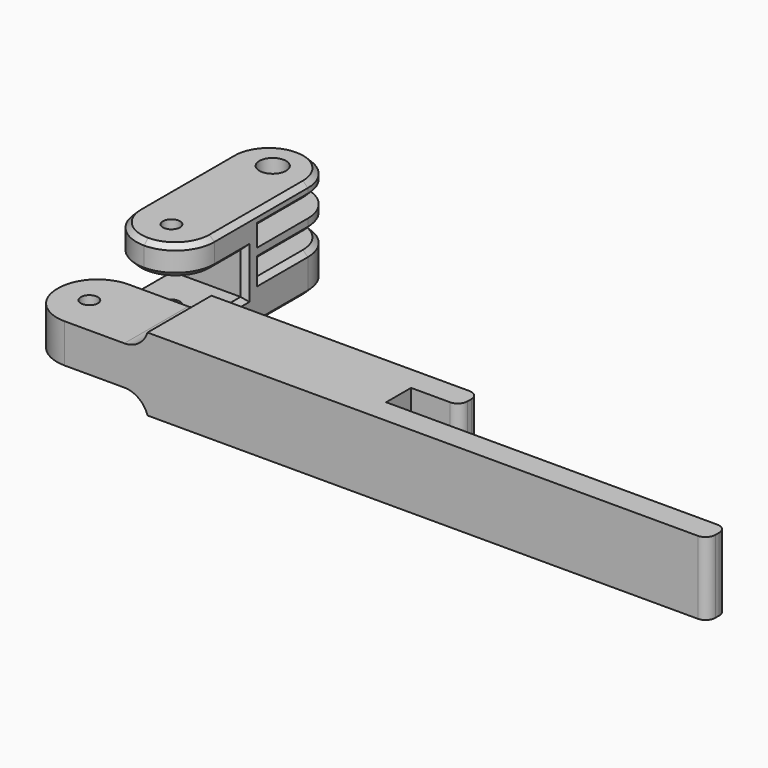
from build123d import *

# Parameters (mm, degrees)
F1_DEPTH     = 15
F3_DEPTH     = 16
F5_R         = 7.99999
F4_R         = 2.75
F4_R_2       = 1.75
F6_DEPTH     = 25
F9_R         = 2
F10_W        = 16.4
F10_H        = 3.5
F11_DEPTH    = 25
F12_R        = 8
F13_R        = 1.75
F14_DEPTH    = 25
F15_T1_DEPTH = 16.4
F16_R        = 2.75
F16_R_2      = 1.75
F17_DEPTH    = 3
F18_SIZE     = 1


# Not quite as in the source:
# - a fillet or chamfer that OpenCascade refuses, or shapes differently, is made with other operations: its cross-section is extruded or revolved along the edge and cut away or added
# - a fillet or chamfer is up to 0.001 mm smaller than in the source, because OpenCascade refuses the exact size
# - a feature of the source that left no trace in its solid (it failed there, or was rolled back) is left out
# - a feature names something its author has since deleted; it is built from what else it names


with BuildPart() as f1:
    # F0 (on Top) → F1 (new body)
    with BuildSketch(Plane.XY):
        Polygon((-2.0918029547, -10.391625925), (-2.0918029547, -3.991625925), (7.9081970453, -3.991625925), (7.9081970453, 1.008374075), (-2.0918029547, 1.008374075), (-72.0918029547, 1.008374075), (-72.0918029547, -15.391625925), (-2.0918029547, -15.391625925), (67.9081970453, -15.391625925), (67.9081970453, -10.391625925), align=None)
    extrude(amount=F1_DEPTH)

    # F9
    f9_edges = [f1.edges().sort_by_distance(p)[0] for p in [
        (7.908197, 1.008374, 7.5),
        (67.908197, -10.391626, 7.5),
        (67.908197, -15.391626, 7.5),
        (7.908197, -3.991626, 7.5),
    ]]
    fillet(f9_edges, radius=F9_R)

    # F10 (on face) → F11 (cut)
    with BuildSketch(Plane(origin=(-72.0918029547, 0, 0), x_dir=(0, -1, 0), z_dir=(-1, 0, 0))):
        with Locations((7.191625925, 1.75)):
            Rectangle(F10_W, F10_H)
        with Locations((7.191625925, 13.25)):
            Rectangle(F10_W, F10_H)
    extrude(amount=-F11_DEPTH, mode=Mode.SUBTRACT)

    # F12
    f12_edges = [f1.edges().sort_by_distance(p)[0] for p in [
        (-72.091803, 1.008374, 7.5),
        (-72.091803, -15.391626, 7.5),
    ]]
    fillet(f12_edges, radius=F12_R)

    # F13 (on face) → F14 (cut)
    with BuildSketch(Plane(origin=(0, 0, 3.5), x_dir=(1, 0, 0), z_dir=(0, 0, -1))):
        with Locations((-65.5918029547, 7.191625925)):
            Circle(F13_R)
    extrude(amount=-F14_DEPTH, mode=Mode.SUBTRACT)

    # F15: fillet of radius 5 on 2 edges, made by hand

    # F15_s2 → F15_t1 (join)
    with BuildSketch(Plane.XZ.offset(-1.008374075)):
        with BuildLine():
            ThreePointArc((-51.8614989618, 3.5), (-48.9034590702, 2.5311288741), (-47.0918029547, 0))
            Line((-47.0918029547, 0), (-47.0918029547, 3.5))
            Line((-47.0918029547, 3.5), (-51.8614989618, 3.5))
        make_face()
        with BuildLine():
            ThreePointArc((-51.8614989618, 11.5), (-48.9034590702, 12.4688711259), (-47.0918029547, 15))
            Line((-47.0918029547, 15), (-47.0918029547, 11.5))
            Line((-47.0918029547, 11.5), (-51.8614989618, 11.5))
        make_face()
    extrude(amount=F15_T1_DEPTH)


with BuildPart() as f3:
    # F2 (on face) → F3 (new body)
    with BuildSketch(Plane(origin=(-72.0918029547, 0, 0), x_dir=(0, -1, 0), z_dir=(-1, 0, 0))):
        Polygon((-25.0802974196, -2.6), (-5, -2.6), (-5, 3.4), (-21, 3.4), (-21, 11.9), (-5, 11.9), (-5, 17.9), (-25, 17.9), (-45, 17.9), (-45, 14.9), (-25, 14.9), (-25, 11.4), (-45, 11.4), (-45, 8.9), (-25, 8.9), (-25, 5.4), (-45, 5.4), (-45, -2.6), align=None)
    extrude(amount=-F3_DEPTH)

    # F5 (radius 8 in the source; OpenCascade refuses exactly that, so slightly less here)
    f5_edges = [f3.edges().sort_by_distance(p)[0] for p in [
        (-56.091803, 45, 1.4),
        (-56.091803, 45, 10.15),
        (-56.091803, 45, 16.4),
        (-72.091803, 45, 1.4),
        (-72.091803, 45, 10.15),
        (-72.091803, 45, 16.4),
        (-72.091803, 5, 0.4),
        (-72.091803, 5, 14.9),
        (-56.091803, 5, 0.4),
        (-56.091803, 5, 14.9),
    ]]
    fillet(f5_edges, radius=F5_R)

    # F4 (on face) → F6 (cut)
    with BuildSketch(Plane(origin=(0, 0, -2.6), x_dir=(1, 0, 0), z_dir=(0, 0, -1))):
        with Locations((-64.0918029547, -38)):
            Circle(F4_R)
        with Locations((-64.0918029547, -12)):
            Circle(F4_R_2)
    extrude(amount=-F6_DEPTH, mode=Mode.SUBTRACT)

    # F16 (on face) → F17 (cut)
    with BuildSketch(Plane(origin=(0, 0, -2.6), x_dir=(1, 0, 0), z_dir=(0, 0, -1))):
        Polygon((-61.9267394452, -34.25), (-66.2568664641, -34.25), (-68.4219299736, -38), (-66.2568664641, -41.75), (-61.9267394452, -41.75), (-59.7616759358, -38), align=None)
        with Locations((-64.0918029547, -38)):
            Circle(F16_R, mode=Mode.SUBTRACT)
        Polygon((-62.2154145798, -8.75), (-65.9681913295, -8.75), (-67.8445797044, -12), (-65.9681913295, -15.25), (-62.2154145798, -15.25), (-60.3390262049, -12), align=None)
        with Locations((-64.0918029547, -12)):
            Circle(F16_R_2, mode=Mode.SUBTRACT)
    extrude(amount=-F17_DEPTH, mode=Mode.SUBTRACT)

    # F18
    f18_edges = [f3.edges().sort_by_distance(p)[0] for p in [
        (-72.091803, 25, 17.9),
        (-72.091803, 25, -2.6),
        (-72.091803, 31.000005, 5.4),
        (-72.091803, 31.000005, 8.9),
        (-72.091803, 31.000005, 14.9),
        (-72.091803, 16.999995, 11.9),
        (-72.091803, 21, 7.65),
        (-72.091803, 16.999995, 3.4),
        (-56.091803, 21, 7.65),
        (-56.091803, 25, 7.15),
        (-56.091803, 25, 13.15),
        (-72.091803, 25, 7.15),
        (-72.091803, 25, 13.15),
        (-64.091803, 45, -2.6),
        (-69.74866, 42.656857, -2.6),
        (-58.434946, 42.656857, -2.6),
        (-56.091803, 25, -2.6),
        (-69.74866, 7.343143, -2.6),
        (-58.434946, 7.343143, -2.6),
        (-64.091803, 5, -2.6),
        (-64.091803, 45, 5.4),
        (-69.74866, 42.656857, 5.4),
        (-58.434946, 42.656857, 5.4),
        (-56.091803, 31.000005, 5.4),
        (-56.091803, 16.999995, 3.4),
        (-56.091803, 31.000005, 8.9),
        (-56.091803, 16.999995, 11.9),
        (-56.091803, 25, 17.9),
        (-56.091803, 31.000005, 14.9),
        (-69.74866, 7.343143, 3.4),
        (-58.434946, 7.343143, 3.4),
        (-64.091803, 5, 3.4),
        (-64.091803, 45, 8.9),
        (-69.74866, 42.656857, 8.9),
        (-58.434946, 42.656857, 8.9),
        (-64.091803, 5, 11.9),
        (-69.74866, 7.343143, 11.9),
        (-58.434946, 7.343143, 11.9),
        (-69.74866, 7.343143, 17.9),
        (-64.091803, 5, 17.9),
        (-58.434946, 7.343143, 17.9),
        (-69.74866, 42.656857, 17.9),
        (-58.434946, 42.656857, 17.9),
        (-64.091803, 45, 17.9),
        (-69.74866, 42.656857, 14.9),
        (-64.091803, 45, 14.9),
        (-58.434946, 42.656857, 14.9),
    ]]
    chamfer(f18_edges, length=F18_SIZE)


solid = Compound([f1.part, f3.part])
